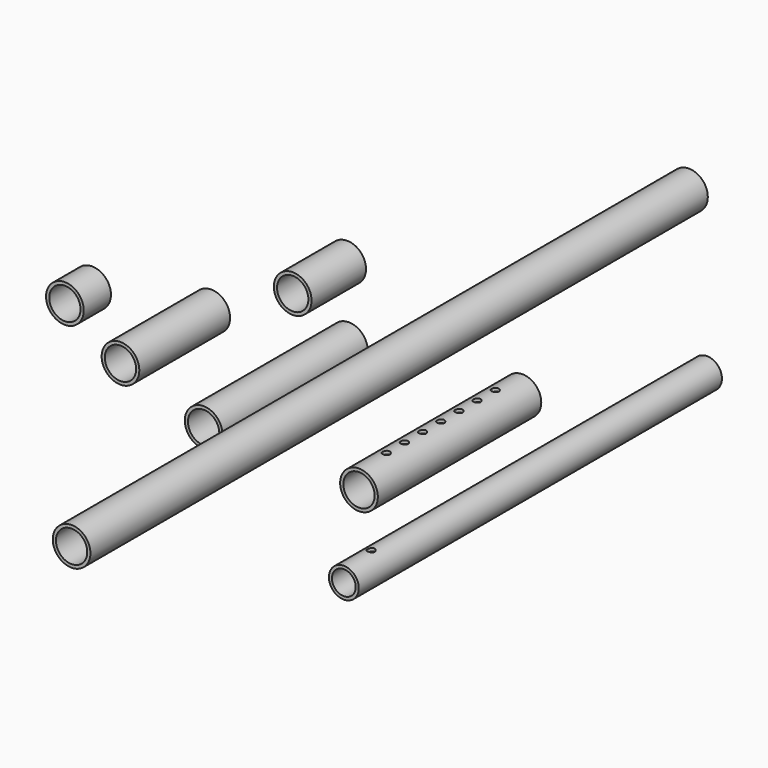
from build123d import *

# Parameters (mm, degrees)
F0_R      = 21.082
F0_R_2    = 17.526
F1_DEPTH  = 431.8
F2_R      = 21.082
F2_R_2    = 17.526
F3_DEPTH  = 114.3
F4_R      = 16.7005
F4_R_2    = 13.3223
F5_DEPTH  = 254
F6_R      = 16.7005
F6_R_2    = 13.3223
F7_DEPTH  = 436.5625
F8_R      = 21.082
F8_R_2    = 17.526
F9_DEPTH  = 38.1
F11_D     = 8.2
F11_2_D   = 8.2
F12_R     = 21.082
F12_R_2   = 17.526
F13_DEPTH = 101.6
F14_R     = 21.082
F14_R_2   = 17.526
F15_DEPTH = 63.5
F16_R     = 21.082
F16_R_2   = 17.526
F17_DEPTH = 19.05


# Not quite as in the source:
# - a feature names something its author has since deleted; it is built from what else it names


with BuildPart() as f1:
    # F0 (on Front) → F1 (new body, symmetric)
    with BuildSketch(Plane.XZ):
        Circle(F0_R)
        Circle(F0_R_2, mode=Mode.SUBTRACT)
    extrude(amount=F1_DEPTH, both=True)


with BuildPart() as f3:
    # F2 (on Front) → F3 (new body, symmetric)
    with BuildSketch(Plane.XZ):
        with Locations((67.6279887557, -51.4777824283)):
            Circle(F2_R)
        with Locations((67.6279887557, -51.4777824283)):
            Circle(F2_R_2, mode=Mode.SUBTRACT)
    extrude(amount=F3_DEPTH, both=True)

    # F11 (through all)
    with Locations(Plane.XY):
        with Locations((67.6279887557, 76.2), (67.6279887557, 50.8), (67.6279887557, 25.4), (162.4108552933, -215.9), (67.6279887557, 0), (67.6279887557, -25.4), (67.6279887557, -50.8), (67.6279887557, -76.2)):
            Hole(F11_D / 2)


with BuildPart() as f5:
    # F4 (on Front) → F5 (new body, symmetric)
    with BuildSketch(Plane.XZ):
        with Locations((162.4108552933, -55.2805289626)):
            Circle(F4_R)
        with Locations((162.4108552933, -55.2805289626)):
            Circle(F4_R_2, mode=Mode.SUBTRACT)
    extrude(amount=F5_DEPTH, both=True)

    # F11#2 (through all)
    with Locations(Plane.XY):
        with Locations((67.6279887557, 76.2), (67.6279887557, 50.8), (67.6279887557, 25.4), (162.4108552933, -215.9), (67.6279887557, 0), (67.6279887557, -25.4), (67.6279887557, -50.8), (67.6279887557, -76.2)):
            Hole(F11_2_D / 2)


with BuildPart() as f7:
    # F6 (on Front) → F7 (new body, symmetric)
    with BuildSketch(Plane.XZ):
        with Locations((249.0000277758, -55.3956031799)):
            Circle(F6_R)
        with Locations((249.0000277758, -55.3956031799)):
            Circle(F6_R_2, mode=Mode.SUBTRACT)
    extrude(amount=F7_DEPTH, both=True)


with BuildPart() as f9:
    # F8 (on Front) → F9 (new body, symmetric)
    with BuildSketch(Plane.XZ):
        with Locations((-67.5115138292, 67.0171454549)):
            Circle(F8_R)
        with Locations((-67.5115138292, 67.0171454549)):
            Circle(F8_R_2, mode=Mode.SUBTRACT)
    extrude(amount=F9_DEPTH, both=True)


with BuildPart() as f13:
    # F12 (on Front) → F13 (new body, symmetric)
    with BuildSketch(Plane.XZ):
        with Locations((-116.3877546787, -55.0170429051)):
            Circle(F12_R)
        with Locations((-116.3877546787, -55.0170429051)):
            Circle(F12_R_2, mode=Mode.SUBTRACT)
    extrude(amount=F13_DEPTH, both=True)


with BuildPart() as f15:
    # F14 (on Front) → F15 (new body, symmetric)
    with BuildSketch(Plane.XZ):
        with Locations((-239.9288862944, -47.454290092)):
            Circle(F14_R)
        with Locations((-239.9288862944, -47.454290092)):
            Circle(F14_R_2, mode=Mode.SUBTRACT)
    extrude(amount=F15_DEPTH, both=True)


with BuildPart() as f17:
    # F16 (on Front) → F17 (new body, symmetric)
    with BuildSketch(Plane.XZ):
        with Locations((-337.6949429512, -38.3744239807)):
            Circle(F16_R)
        with Locations((-337.6949429512, -38.3744239807)):
            Circle(F16_R_2, mode=Mode.SUBTRACT)
    extrude(amount=F17_DEPTH, both=True)


solid = Compound([f1.part, f3.part, f5.part, f9.part, f13.part, f15.part, f17.part])
